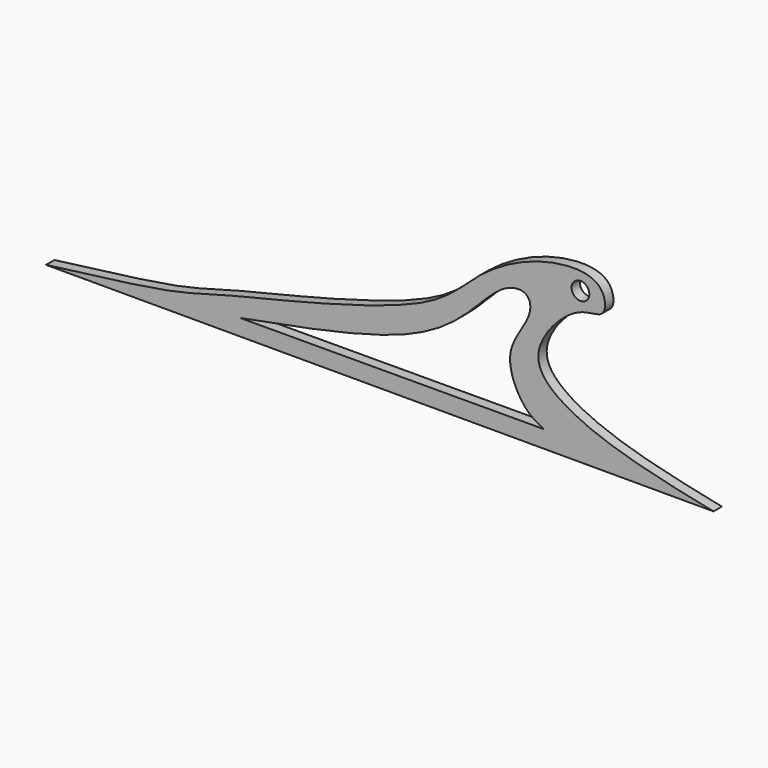
from build123d import *

# Parameters (mm, degrees)
F1_DEPTH = 3
F2_R     = 2.54
F3_DEPTH = 25.4


# Not quite as in the source:
# - a feature names something its author has since deleted; it is built from what else it names


with BuildPart() as f1:
    # F0 (on Front) → F1 (new body)
    with BuildSketch(Plane.XZ):
        with BuildLine():
            add(Edge.make_bspline(
                [(-203.1916106619, 0.1913178712), (-162.7239087005, 5.1608725361), (-168.3456273381, 6.283736461), (-92.3994399685, 22.5296334539), (-80.7657565229, 38.1452471787), (-62.1132756355, 48.6899093444), (-43.455198512, 49.3507332073), (-42.4219565639, 37.9703684819), (-51.7510128272, 40.0764215485), (-67.0289361999, 23.0552343494), (-54.1253670283, 11.4212539718), (-33.5917608798, 4.6260542829), (-19.3620556884, 1.6860036467), (-12.1274217963, 0.1913178712)],
                knots=[0, 0, 0, 0, 0.140678246, 0.2947426936, 0.384172525, 0.4744748119, 0.5534022467, 0.6036077636, 0.6566936259, 0.7416412148, 0.8136119401, 0.9066577692, 1, 1, 1, 1], degree=3))
            Line((-203.1916106619, 0.1913178712), (-12.1274217963, 0.1913178712))
        make_face()
        with BuildLine():
            Line((-60.6277957559, 5.1366542466), (-147.653222084, 4.8829359002))
            add(Edge.make_bspline(
                [(-147.653222084, 4.8829359002), (-130.3589714209, 8.0826541566), (-101.4779807426, 13.426108171), (-83.1679275212, 25.4745889426), (-72.9717774064, 38.0426898937), (-64.86592143, 38.4744537878), (-63.7926032387, 31.5969719498), (-73.3136713805, 21.6552008441), (-66.7268411849, 8.0515220574), (-62.4116540428, 5.9891993145), (-60.6277957559, 5.1366542466)],
                knots=[0, 0, 0, 0, 0.2319631686, 0.3873730202, 0.5186490792, 0.599825011, 0.674025894, 0.7932480048, 0.9145306454, 1, 1, 1, 1], degree=3))
        make_face(mode=Mode.SUBTRACT)
    extrude(amount=F1_DEPTH)

    # F2 (on Front) → F3 (cut)
    with BuildSketch(Plane.XZ):
        with Locations((-50.2274217963, 43.3713178712)):
            Circle(F2_R)
    extrude(amount=F3_DEPTH, mode=Mode.SUBTRACT)


solid = f1.part
